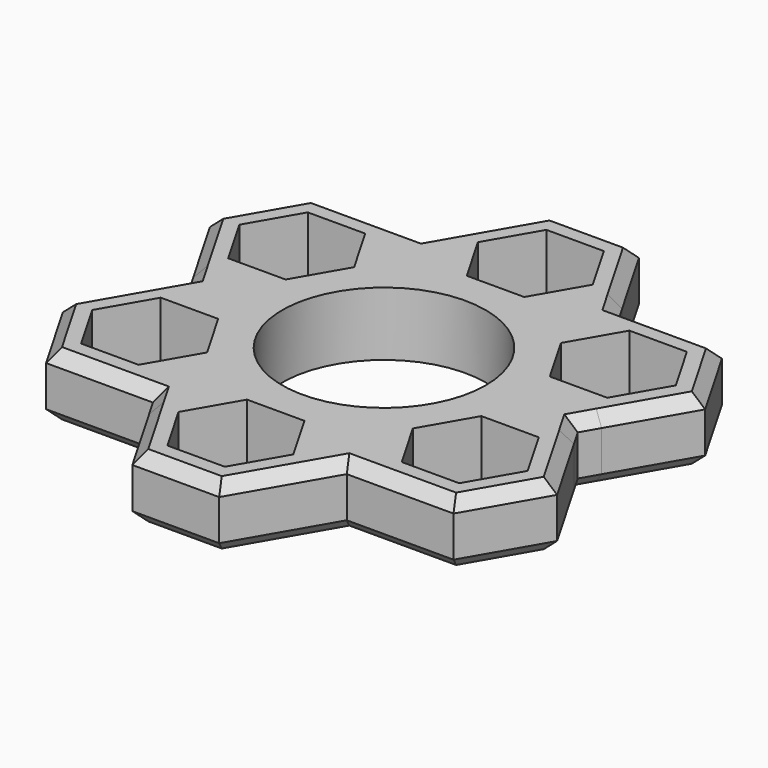
from build123d import *

# Parameters (mm, degrees)
F1_DEPTH = 6.9977
F2_R     = 11.176
F3_DEPTH = 6.9977
F4_SIZE  = 1.27


# Not quite as in the source:
# - a feature names something its author has since deleted; it is built from what else it names


with BuildPart() as f1:
    # F0 (on Top) → F1 (new body)
    with BuildSketch(Plane.XY):
        Polygon((-1.27, 12.7), (1.27, 12.7), (5.4871048633, 12.7), (6.9125849394, 15.169003917), (7.0907659214, 15.4776224307), (9.8865139145, 20.32), (5.1204874424, 28.575), (-4.411565502, 28.575), (-9.1775919741, 20.32), (-4.7781829229, 12.7), align=None)
        Polygon((6.6602806103, 20.32), (3.5073707902, 14.859), (-2.7984488498, 14.859), (-5.9513586699, 20.32), (-2.7984488498, 25.781), (3.5073707902, 25.781), align=None, mode=Mode.SUBTRACT)
        Polygon((6.9125849394, 15.169003917), (5.4871048633, 12.7), (7.3323484187, 12.7), (8.4322006815, 10.795), (12.8316097327, 18.415), (10.9863661773, 18.415), (9.8865139145, 20.32), (7.0907659214, 15.4776224307), align=None)
        Polygon((-7.3323484187, 12.7), (-4.7781829229, 12.7), (-9.1775919741, 20.32), (-10.3250266623, 18.3325848218), (-12.8789355329, 18.3325848218), (-8.4796547943, 10.7128070657), align=None)
        Polygon((12.8316097327, 18.415), (8.4322006815, 10.795), (11.6335226281, 5.2501477372), (13.5648445746, 1.905), (16.3276362049, 1.905), (18.8676362049, 1.905), (22.3636626771, 1.905), (27.1296891492, 10.16), (22.3636626771, 18.415), align=None)
        Polygon((20.7505460249, 4.699), (14.4447263849, 4.699), (11.2918165648, 10.16), (14.4447263849, 15.621), (20.7505460249, 15.621), (23.903455845, 10.16), align=None, mode=Mode.SUBTRACT)
        Polygon((-9.8614826635, 8.3194109889), (-8.4796547943, 10.7128070657), (-12.8789355329, 18.3325848218), (-22.4109884772, 18.3325848218), (-27.1770149494, 10.0775848218), (-22.4109884772, 1.8225848218), (-13.612427, 1.8225848218), (-11.1783483187, 6.0385327673), align=None)
        Polygon((-14.492052185, 15.5385848218), (-11.339142365, 10.0775848218), (-14.492052185, 4.6165848218), (-20.7978718251, 4.6165848218), (-23.9507816452, 10.0775848218), (-20.7978718251, 15.5385848218), align=None, mode=Mode.SUBTRACT)
        Polygon((16.3276362049, 1.905), (13.5648445746, 1.905), (14.6646968374, 0), (13.5648445746, -1.905), (22.3636626771, -1.905), (21.2638104143, 0), (22.3636626771, 1.905), (18.8676362049, 1.905), align=None)
        Polygon((-14.6646968374, 0), (-13.612427, 1.8225848218), (-22.4109884772, 1.8225848218), (-21.311264527, -0.0821929343), (-22.3636626771, -1.905), (-19.9342235854, -1.905), (-17.3764717744, -1.905), (-13.5648445746, -1.905), align=None)
        Polygon((22.3636626771, -1.905), (13.5648445746, -1.905), (10.3635226281, -7.4498522628), (8.4322006815, -10.795), (9.8135964967, -13.1876477372), (11.0835964967, -15.3873522628), (12.8316097327, -18.415), (22.3636626771, -18.415), (27.1296891492, -10.16), align=None)
        Polygon((14.4447263849, -15.621), (11.2918165648, -10.16), (14.4447263849, -4.699), (20.7505460249, -4.699), (23.903455845, -10.16), (20.7505460249, -15.621), align=None, mode=Mode.SUBTRACT)
        Polygon((-11.6335226281, -5.2501477372), (-13.5648445746, -1.905), (-17.3764717744, -1.905), (-19.9342235854, -1.905), (-22.3636626771, -1.905), (-27.1296891492, -10.16), (-22.3636626771, -18.415), (-12.8316097327, -18.415), (-8.4322006815, -10.795), (-10.3635226281, -7.4498522628), align=None)
        Polygon((-20.7505460249, -4.699), (-14.4447263849, -4.699), (-11.2918165648, -10.16), (-14.4447263849, -15.621), (-20.7505460249, -15.621), (-23.903455845, -10.16), align=None, mode=Mode.SUBTRACT)
        Polygon((9.8135964967, -13.1876477372), (8.4322006815, -10.795), (7.3323484187, -12.7), (5.1326438931, -12.7), (9.5320529443, -20.32), (4.7660264722, -28.575), (10.6457036946, -18.415), (12.8316097327, -18.415), (11.0835964967, -15.3873522628), align=None)
        Polygon((9.5320529443, -20.32), (5.1326438931, -12.7), (1.27, -12.7), (-1.27, -12.7), (-5.1326438931, -12.7), (-6.5140397082, -15.0926477372), (-7.7840397082, -17.2923522628), (-9.5320529443, -20.32), (-4.7660264722, -28.575), (4.7660264722, -28.575), align=None)
        Polygon((-6.3058196401, -20.32), (-3.15290982, -14.859), (3.15290982, -14.859), (6.3058196401, -20.32), (3.15290982, -25.781), (-3.15290982, -25.781), align=None, mode=Mode.SUBTRACT)
        Polygon((-7.3323484187, -12.7), (-8.4322006815, -10.795), (-12.8316097327, -18.415), (-10.6319052071, -18.415), (-9.5320529443, -20.32), (-7.7840397082, -17.2923522628), (-6.5140397082, -15.0926477372), (-5.1326438931, -12.7), align=None)
        Polygon((5.4871048633, 12.7), (1.27, 12.7), (-1.27, 12.7), (-4.7781829229, 12.7), (-4.411565502, 12.065), (-2.0086818804, 12.065), (1.267424375, 12.065), (5.1204874424, 12.065), align=None)
        Polygon((-12.8316097327, -1.905), (-13.5648445746, -1.905), (-11.6335226281, -5.2501477372), (-11.0835964967, -4.9326477372), align=None)
        Polygon((1.27, -12.7), (5.1326438931, -12.7), (4.7660264722, -12.065), (1.27, -12.065), (-1.27, -12.065), (-4.7660264722, -12.065), (-5.1326438931, -12.7), (-1.27, -12.7), align=None)
        Polygon((9.8135964967, -7.1323522628), (10.3635226281, -7.4498522628), (11.5783918417, -5.2183179628), (11.0835964967, -4.9326477372), align=None)
        Polygon((11.0835964967, 4.9326477372), (11.6335226281, 5.2501477372), (10.3083918417, 7.4180224884), (9.8135964967, 7.1323522628), align=None)
        Polygon((-9.3113640632, 8.0017998669), (-9.8614826635, 8.3194109889), (-11.1783483187, 6.0385327673), (-10.6282297184, 5.7209216453), align=None)
        Polygon((11.6335226281, 5.2501477372), (8.4322006815, 10.795), (8.0655832606, 10.16), (9.8135964967, 7.1323522628), (10.3083918417, 7.4180224884), align=None)
        Polygon((10.3635226281, -7.4498522628), (13.5648445746, -1.905), (12.8316097327, -1.905), (11.0835964967, -4.9326477372), (11.5783918417, -5.2183179628), align=None)
    extrude(amount=F1_DEPTH)

    # F2 (on Top) → F3 (join)
    with BuildSketch(Plane.XY):
        Polygon((7.6989658396, 13.335), (-7.6989658396, 13.335), (-15.3979316793, 0), (-7.6989658396, -13.335), (7.6989658396, -13.335), (15.3979316793, 0), align=None)
        Circle(F2_R, mode=Mode.SUBTRACT)
    extrude(amount=F3_DEPTH)

    # F4
    f4_edges = [f1.edges().sort_by_distance(p)[0] for p in [
        (-16.497784, -18.415, 6.9977),
        (-16.497784, -18.415, 0),
        (-7.698966, -23.495, 6.9977),
        (-7.698966, -23.495, 0),
        (0, -28.575, 6.9977),
        (0, -28.575, 0),
        (7.705865, -23.495, 0),
        (7.705865, -23.495, 6.9977),
        (16.504683, -18.415, 0),
        (16.504683, -18.415, 6.9977),
        (24.746676, -14.2875, 6.9977),
        (24.746676, -14.2875, 0),
        (24.19675, 5.08, 0),
        (24.19675, 5.08, 6.9977),
        (24.746676, 14.2875, 6.9977),
        (24.746676, 14.2875, 0),
        (16.675014, 18.415, 0),
        (16.675014, 18.415, 6.9977),
        (8.053427, 23.495, 0),
        (8.053427, 23.495, 6.9977),
        (0.354461, 28.575, 0),
        (0.354461, 28.575, 6.9977),
        (-7.368296, 23.453792, 6.9977),
        (-7.368296, 23.453792, 0),
        (-16.368008, 18.332585, 0),
        (-16.368008, 18.332585, 6.9977),
        (-24.794002, 14.205085, 0),
        (-24.794002, 14.205085, 6.9977),
        (-24.24414, 4.997696, 6.9977),
        (-24.24414, 4.997696, 0),
        (-24.220477, -5.121096, 0),
        (-24.220477, -5.121096, 6.9977),
        (-24.746676, -14.2875, 6.9977),
        (-24.746676, -14.2875, 0),
        (24.19675, -5.08, 0),
        (24.19675, -5.08, 6.9977),
    ]]
    chamfer(f4_edges, length=F4_SIZE)


solid = f1.part
